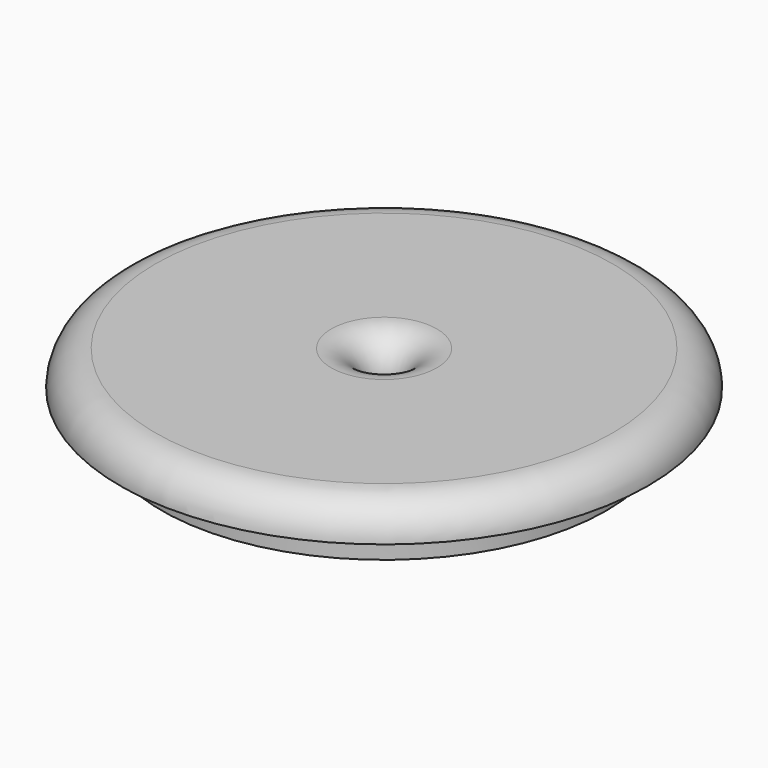
from build123d import *

# Parameters (mm, degrees)
F0_R     = 19.05
F0_R_2   = 16.1925
F0_R_3   = 1.27
F1_DEPTH = 2.54
F2_DEPTH = 2.54
F2_TAPER = 3
F3_R     = 2.53999
F4_R     = 2.53999
F4_2_R   = 2.53999


# Not quite as in the source:
# - a fillet or chamfer is up to 0.001 mm smaller than in the source, because OpenCascade refuses the exact size


with BuildPart() as f1:
    # F0 (on Top) → F1 (new body)
    with BuildSketch(Plane.XY):
        Circle(F0_R)
        Circle(F0_R_2, mode=Mode.SUBTRACT)
        Circle(F0_R_2)
        Circle(F0_R_3, mode=Mode.SUBTRACT)
    extrude(amount=F1_DEPTH)

    # F3 (radius 2.54 in the source; OpenCascade refuses exactly that, so slightly less here)
    f3_edges = [f1.edges().sort_by_distance(p)[0] for p in [
        (-19.05, 0, 2.54),
    ]]
    fillet(f3_edges, radius=F3_R)

    # F4 (radius 2.54 in the source; OpenCascade refuses exactly that, so slightly less here)
    f4_edges = [f1.edges().sort_by_distance(p)[0] for p in [
        (-1.27, 0, 2.54),
    ]]
    fillet(f4_edges, radius=F4_R)


with BuildPart() as f2:
    # F0 (on Top) → F2 (new body)
    with BuildSketch(Plane.XY):
        Circle(F0_R_2)
        Circle(F0_R_3, mode=Mode.SUBTRACT)
    extrude(amount=-F2_DEPTH, taper=F2_TAPER)

    # F4#2 (radius 2.54 in the source; OpenCascade refuses exactly that, so slightly less here)
    f4_2_edges = [f2.edges().sort_by_distance(p)[0] for p in [
        (-1.403116, 0, -2.54),
    ]]
    fillet(f4_2_edges, radius=F4_2_R)


solid = Compound([f1.part, f2.part])
